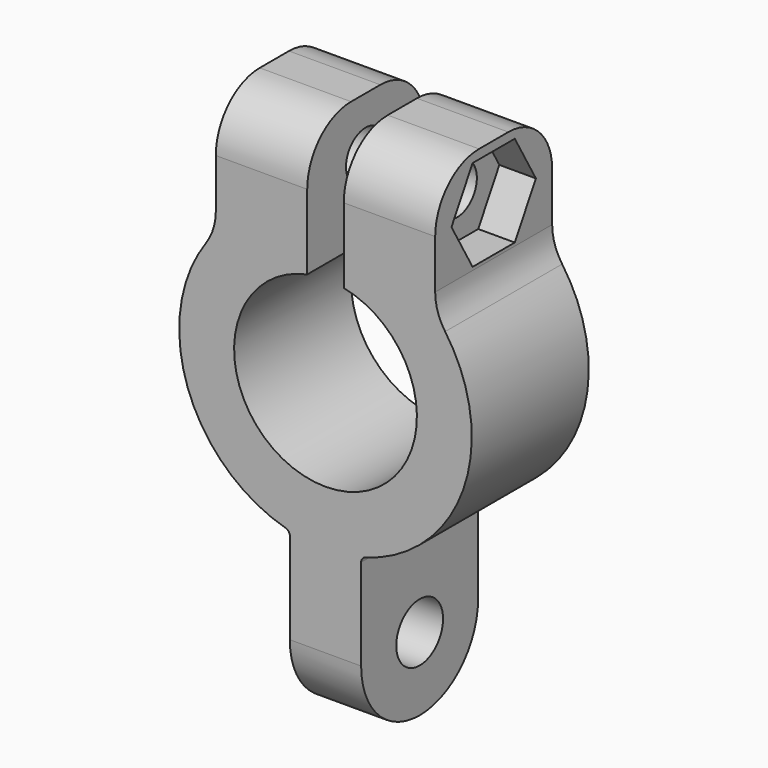
from build123d import *

# Parameters (mm, degrees)
F1_DEPTH = 4
F2_R     = 1.35
F3_DEPTH = 25
F4_DEPTH = 2
F5_R     = 1.6
F6_DEPTH = 25
F7_SIZE  = 1.35
F8_R     = 3
F9_R     = 3.99999


# Not quite as in the source:
# - a fillet or chamfer is up to 0.001 mm smaller than in the source, because OpenCascade refuses the exact size
# - a feature names something its author has since deleted; it is built from what else it names


with BuildPart() as f1:
    # F0 (on Front) → F1 (new body, symmetric)
    with BuildSketch(Plane.XZ):
        with BuildLine():
            ThreePointArc((1, 4.8989794856), (0, -5), (-1, 4.8989794856))
            Line((-1, 4.8989794856), (-1, 12))
            Line((-1, 12), (-6, 12))
            Line((-6, 12), (-6, 5.2915026221))
            ThreePointArc((-6, 5.2915026221), (-7.6747647209, -2.257872113), (-2.1786734922, -7.6976218285))
            ThreePointArc((-2.1786734922, -7.6976218285), (-2.0136051919, -7.8104451764), (-1.95, -8))
            Line((-1.95, -8), (-1.95, -17))
            Line((-1.95, -17), (1.95, -17))
            Line((1.95, -17), (1.95, -8))
            ThreePointArc((1.95, -8), (2.0136051919, -7.8104451764), (2.1786734922, -7.6976218285))
            ThreePointArc((2.1786734922, -7.6976218285), (7.6747647209, -2.257872113), (6, 5.2915026221))
            Line((6, 5.2915026221), (6, 12))
            Line((6, 12), (1, 12))
            Line((1, 12), (1, 4.8989794856))
        make_face()
    extrude(amount=F1_DEPTH, both=True)

    # F2 (on face) → F3 (cut)
    with BuildSketch(Plane.YZ.offset(6)):
        with Locations((0, 9)):
            Circle(F2_R)
    extrude(amount=-F3_DEPTH, mode=Mode.SUBTRACT)

    # F2 (on face) → F4 (cut)
    with BuildSketch(Plane.YZ.offset(6)):
        Polygon((2.8867513459, 9), (1.443375673, 11.5), (-1.443375673, 11.5), (-2.8867513459, 9), (-1.443375673, 6.5), (1.443375673, 6.5), align=None)
        with Locations((0, 9)):
            Circle(F2_R, mode=Mode.SUBTRACT)
    extrude(amount=-F4_DEPTH, mode=Mode.SUBTRACT)

    # F5 (on face) → F6 (cut)
    with BuildSketch(Plane.YZ.offset(1.95)):
        with Locations((0, -13)):
            Circle(F5_R)
    extrude(amount=-F6_DEPTH, mode=Mode.SUBTRACT)

    # F7
    f7_edges = [f1.edges().sort_by_distance(p)[0] for p in [
        (-6, -1.35, 9),
    ]]
    chamfer(f7_edges, length=F7_SIZE)

    # F8
    f8_edges = [f1.edges().sort_by_distance(p)[0] for p in [
        (-3.5, -4, 12),
        (-3.5, 4, 12),
        (3.5, 4, 12),
        (3.5, -4, 12),
        (6, 0, 5.291503),
        (-6, 0, 5.291503),
    ]]
    fillet(f8_edges, radius=F8_R)

    # F9 (radius 4 in the source; OpenCascade refuses exactly that, so slightly less here)
    f9_edges = [f1.edges().sort_by_distance(p)[0] for p in [
        (0, -4, -17),
        (0, 4, -17),
    ]]
    fillet(f9_edges, radius=F9_R)


solid = f1.part
